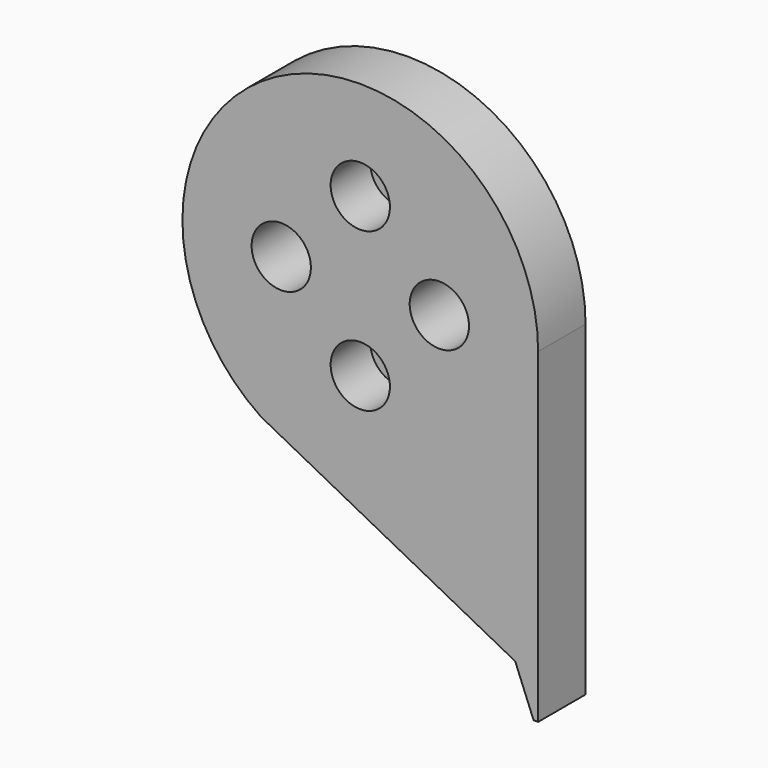
from build123d import *

# Parameters (mm, degrees)
F1_DEPTH    = 6
F2_SIZE2    = 4.99999
F2_SIZE     = 1.99999
F3_T4_DEPTH = 15.7736618076
F3_T9_DEPTH = 15.7736618076
F4_T4_DEPTH = 8.4627924491
F4_T9_DEPTH = 8.4627924491
F5_R        = 13.3817573781
F5_R_2      = 3
F5_R_3      = 2
F6_DEPTH    = 8
F7_DEPTH    = 8.001
F8_DEPTH    = 5


# Not quite as in the source:
# - a fillet or chamfer that OpenCascade refuses, or shapes differently, is made with other operations: its cross-section is extruded or revolved along the edge and cut away or added
# - a fillet or chamfer is up to 0.001 mm smaller than in the source, because OpenCascade refuses the exact size


with BuildPart() as f1:
    # F0 (on Front) → F1 (new body)
    with BuildSketch(Plane.XZ):
        with BuildLine():
            ThreePointArc((-6.5061441265, -16.7830297803), (10.1707769055, -14.8511042397), (18, 0))
            ThreePointArc((18, 0), (-8.4642142433, 15.8857507611), (-10.0396752493, -14.9400442064))
            Line((-10.0396752493, -14.9400442064), (-6.5061441265, -16.7830297803))
        make_face()
        with BuildLine():
            Line((18, -33), (18, 0))
            ThreePointArc((18, 0), (10.1707769055, -14.8511042397), (-6.5061441265, -16.7830297803))
            Line((-6.5061441265, -16.7830297803), (15, -28))
            Line((15, -28), (15, -33))
            Line((15, -33), (18, -33))
        make_face()
    extrude(amount=F1_DEPTH)

    # F2 (size 2 and 5 in the source; OpenCascade refuses exactly that, so slightly less here)
    f2_edges = [f1.edges().sort_by_distance(p)[0] for p in [
        (15, -3, -33),
    ]]
    f2_side = f1.faces().sort_by_distance((16.5, -3, -33))[0]
    chamfer(f2_edges, length=F2_SIZE, length2=F2_SIZE2, reference=f2_side)

    # F3: chamfer of 0.5 x 2 on 2 edges, made by hand


with BuildPart() as f3_tool2:
    # F3_s3 → F3_t4 (new body)
    with BuildSketch(Plane(origin=(15.653192591, 0, -39.1330988771), x_dir=(0, 1, 0), z_dir=(-0.3713897159, 0, 0.9284770751))):
        Polygon((0, -4.0282403683), (-2, -3.5282403683), (0, -3.5282403683), align=None)
    extrude(amount=F3_T4_DEPTH)

    split(bisect_by=Plane(origin=(-8.2729096879, 0, -15.8615369933), x_dir=(0, 1, 0), z_dir=(-0.4624484745, 0, -0.8866461574)), keep=Keep.TOP)


with BuildPart() as f1_1:
    add(f1.part)

    # F3_t1: cut F3_tool2
    add(f3_tool2.part, mode=Mode.SUBTRACT)


with BuildPart() as f3_tool7:
    # F3_s8 → F3_t9 (new body)
    with BuildSketch(Plane(origin=(15.653192591, 0, -39.1330988771), x_dir=(0, 1, 0), z_dir=(-0.3713897159, 0, 0.9284770751))):
        Polygon((-4, -3.5282403683), (-6, -4.0282403683), (-6, -3.5282403683), align=None)
    extrude(amount=F3_T9_DEPTH)

    split(bisect_by=Plane(origin=(-8.2729096879, 0, -15.8615369933), x_dir=(0, 1, 0), z_dir=(-0.4624484745, 0, -0.8866461574)), keep=Keep.TOP)


with BuildPart() as f1_2:
    add(f1_1.part)

    # F3_t6: cut F3_tool7
    add(f3_tool7.part, mode=Mode.SUBTRACT)

    # F4: fillet of radius 5 on 2 edges, made by hand


with BuildPart() as f4_tool2:
    # F4_s3 → F4_t4 (new body)
    with BuildSketch(Plane(origin=(14.2956017442, 0, -35.739111578), x_dir=(0, 1, 0), z_dir=(-0.3713897159, 0, 0.9284770751))):
        with BuildLine():
            ThreePointArc((-1.4028500029, -3.6775278676), (-2.0046118096, -3.5657025849), (-2.615528128, -3.5282403683))
            Line((-2.615528128, -3.5282403683), (-2, -3.5282403683))
            Line((-2, -3.5282403683), (-1.4028500029, -3.6775278676))
        make_face()
    extrude(amount=F4_T4_DEPTH)

    split(bisect_by=Plane(origin=(-8.2729096879, 0, -15.8615369933), x_dir=(0, 1, 0), z_dir=(-0.4624484745, 0, -0.8866461574)), keep=Keep.TOP)


with BuildPart() as f1_3:
    add(f1_2.part)

    # F4_t1: cut F4_tool2
    add(f4_tool2.part, mode=Mode.SUBTRACT)


with BuildPart() as f4_tool7:
    # F4_s8 → F4_t9 (new body)
    with BuildSketch(Plane(origin=(14.2956017442, 0, -35.739111578), x_dir=(0, 1, 0), z_dir=(-0.3713897159, 0, 0.9284770751))):
        with BuildLine():
            ThreePointArc((-4.5971499971, -3.6775278676), (-3.9953881904, -3.5657025849), (-3.384471872, -3.5282403683))
            Line((-3.384471872, -3.5282403683), (-4, -3.5282403683))
            Line((-4, -3.5282403683), (-4.5971499971, -3.6775278676))
        make_face()
    extrude(amount=F4_T9_DEPTH)

    split(bisect_by=Plane(origin=(-8.2729096879, 0, -15.8615369933), x_dir=(0, 1, 0), z_dir=(-0.4624484745, 0, -0.8866461574)), keep=Keep.TOP)


with BuildPart() as f1_4:
    add(f1_3.part)

    # F4_t6: cut F4_tool7
    add(f4_tool7.part, mode=Mode.SUBTRACT)

    # F5 (on face) → F6 (join)
    with BuildSketch(Plane.XZ.offset(6)):
        Circle(F5_R)
        with Locations((0, -8)):
            Circle(F5_R_2, mode=Mode.SUBTRACT)
        with Locations((-8, 0)):
            Circle(F5_R_2, mode=Mode.SUBTRACT)
        with Locations((8, 0)):
            Circle(F5_R_2, mode=Mode.SUBTRACT)
        with Locations((0, 8)):
            Circle(F5_R_2, mode=Mode.SUBTRACT)
        with Locations((0, 8)):
            Circle(F5_R_2)
        with Locations((0, 8)):
            Circle(F5_R_3, mode=Mode.SUBTRACT)
        with Locations((0, -8)):
            Circle(F5_R_2)
        with Locations((0, -8)):
            Circle(F5_R_3, mode=Mode.SUBTRACT)
        with Locations((-8, 0)):
            Circle(F5_R_2)
        with Locations((8, 0)):
            Circle(F5_R_2)
        with Locations((0, 8)):
            Circle(F5_R_3)
        with Locations((0, -8)):
            Circle(F5_R_3)
    extrude(amount=-F6_DEPTH)

    # F5 (on face) → F7 (cut, through all)
    with BuildSketch(Plane.XZ.offset(6)):
        with Locations((-8, 0)):
            Circle(F5_R_2)
        with Locations((0, 8)):
            Circle(F5_R_3)
        with Locations((8, 0)):
            Circle(F5_R_2)
        with Locations((0, -8)):
            Circle(F5_R_3)
    extrude(amount=-F7_DEPTH, mode=Mode.SUBTRACT)

    # F5 (on face) → F8 (cut)
    with BuildSketch(Plane.XZ.offset(6)):
        with Locations((0, 8)):
            Circle(F5_R_2)
        with Locations((0, 8)):
            Circle(F5_R_3, mode=Mode.SUBTRACT)
        with Locations((0, -8)):
            Circle(F5_R_2)
        with Locations((0, -8)):
            Circle(F5_R_3, mode=Mode.SUBTRACT)
    extrude(amount=-F8_DEPTH, mode=Mode.SUBTRACT)


solid = f1_4.part
